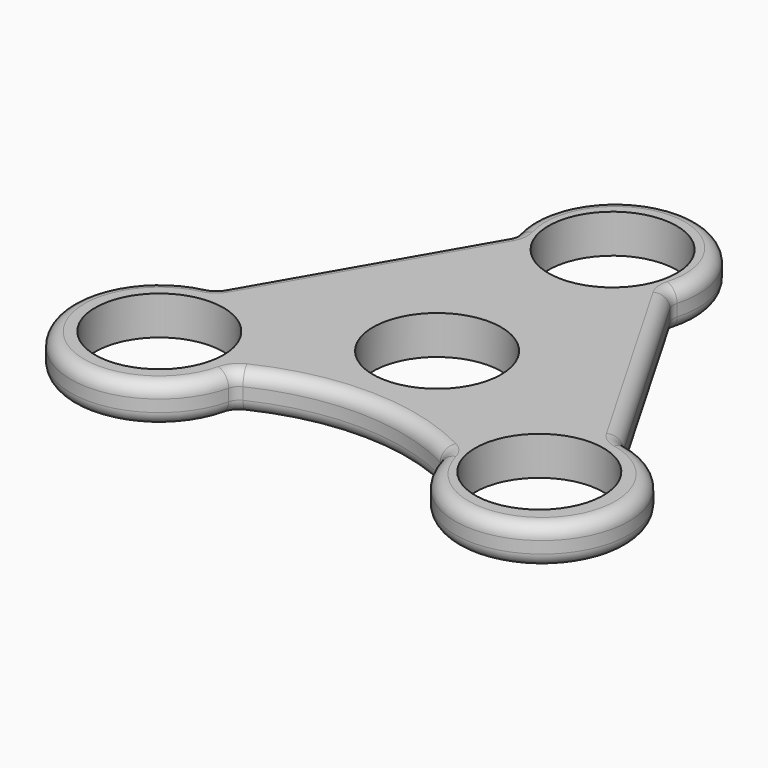
from build123d import *

# Parameters (mm, degrees)
F0_R     = 10.922
F1_DEPTH = 6.604
F2_R     = 2.286


with BuildPart() as f1:
    # F0 (on Top) → F1 (new body)
    with BuildSketch(Plane.XY):
        with BuildLine():
            Line((-13.3873032043, 33.1231516497), (-34.7322359773, -3.8473563972))
            ThreePointArc((-34.7322359773, -3.8473563972), (-43.0701011693, -29.3490933873), (-17.4819467583, -21.2803302039))
            ThreePointArc((-17.4819467583, -21.2803302039), (0.6081285176, -17.0457166579), (18.5540814858, -21.8546195923))
            ThreePointArc((18.5540814858, -21.8546195923), (43.8875031627, -29.0995032663), (34.9920927448, -4.2974415213))
            Line((34.9920927448, -4.2974415213), (13.3533630424, 33.1819377345))
            ThreePointArc((13.3533630424, 33.1819377345), (-0.0588324041, 52.1949153144), (-13.3873032043, 33.1231516497))
        make_face()
        with Locations((-32.3834455885, -18.6965910278)):
            Circle(F0_R, mode=Mode.SUBTRACT)
        Circle(F0_R, mode=Mode.SUBTRACT)
        with BuildLine():
            ThreePointArc((23.643944132, -25.247254986), (28.9311094886, -8.3345709808), (43.3054455885, -18.6965910278))
            ThreePointArc((43.3054455885, -18.6965910278), (35.8980520612, -29.0376560282), (23.7233863792, -25.3519241143))
            ThreePointArc((23.7233863792, -25.3519241143), (23.6835078446, -25.2997090226), (23.643944132, -25.247254986))
        make_face(mode=Mode.SUBTRACT)
        with Locations((0, 37.3931820556)):
            Circle(F0_R, mode=Mode.SUBTRACT)
    extrude(amount=F1_DEPTH)

    # F2
    f2_edges = [f1.edges().sort_by_distance(p)[0] for p in [
        (-17.481947, -21.28033, 3.302),
        (18.554081, -21.85462, 3.302),
        (34.992093, -4.297442, 3.302),
        (-13.387303, 33.123152, 3.302),
        (-34.732236, -3.847356, 3.302),
        (13.353363, 33.181938, 3.302),
        (-0.058832, 52.194915, 0),
        (-0.058832, 52.194915, 6.604),
        (-24.05977, 14.637898, 0),
        (-24.05977, 14.637898, 6.604),
        (-43.070101, -29.349093, 6.604),
        (0.608129, -17.045717, 6.604),
        (43.887503, -29.099503, 6.604),
        (24.172728, 14.442248, 6.604),
        (24.172728, 14.442248, 0),
        (43.887503, -29.099503, 0),
        (0.608129, -17.045717, 0),
        (-43.070101, -29.349093, 0),
    ]]
    fillet(f2_edges, radius=F2_R)


solid = f1.part
